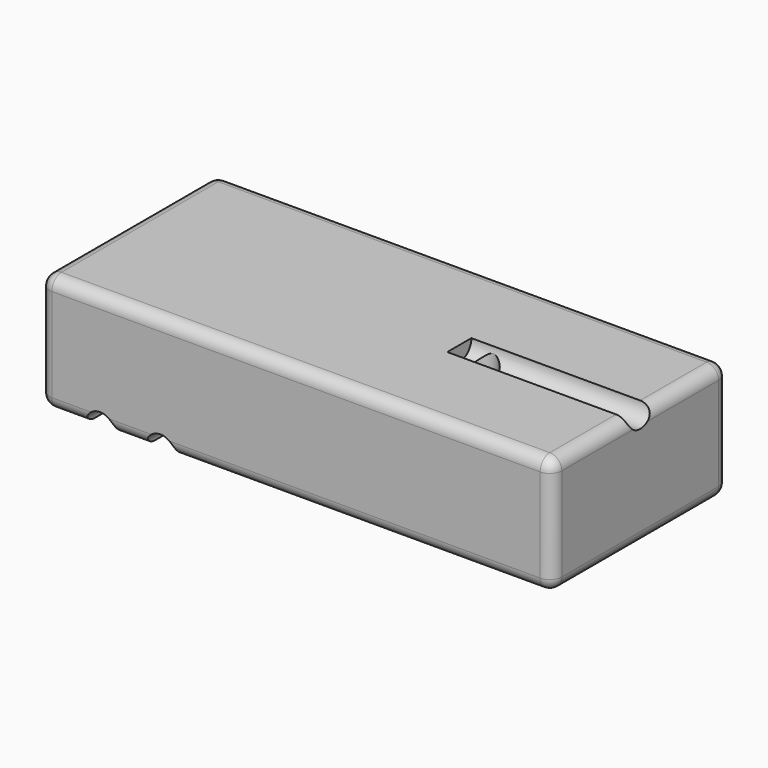
from build123d import *

# Parameters (mm, degrees)
F0_W         = 215.9
F0_H         = 92.71
F1_DEPTH     = 49.53
F3_DEPTH     = 76.2
F5_DEPTH     = 92.71
F6_R         = 5.08
F7_R         = 6.35
F8_DEPTH     = 92.7110001
F9_T1_DEPTH  = 26.67
F9_S5_W      = 5.08
F9_S5_H      = 5.08
F9_T6_DEPTH  = 5.08
F9_S11_W     = 5.08
F9_S11_H     = 5.08
F9_T12_DEPTH = 5.08
F10_R        = 5.588
F11_DEPTH    = 49.5310001


# Not quite as in the source:
# - a fillet or chamfer that OpenCascade refuses, or shapes differently, is made with other operations: its cross-section is extruded or revolved along the edge and cut away or added


with BuildPart() as f1:
    # F0 (on Top) → F1 (new body)
    with BuildSketch(Plane.XY):
        with Locations((107.95, 46.355)):
            Rectangle(F0_W, F0_H)
    extrude(amount=F1_DEPTH)

    # F2 (on face) → F3 (cut)
    with BuildSketch(Plane.YZ.offset(215.9)):
        with BuildLine():
            Line((52.705, 49.53), (40.005, 49.53))
            ThreePointArc((40.005, 49.53), (46.355, 43.18), (52.705, 49.53))
        make_face()
    extrude(amount=-F3_DEPTH, mode=Mode.SUBTRACT)

    # F4 (on face) → F5 (cut, through all)
    with BuildSketch(Plane.XZ):
        with BuildLine():
            Line((19.05, 0), (31.75, 0))
            ThreePointArc((31.75, 0), (25.4, 6.35), (19.05, 0))
        make_face()
    extrude(amount=-F5_DEPTH, mode=Mode.SUBTRACT)

    # F6
    f6_edges = [f1.edges().sort_by_distance(p)[0] for p in [
        (107.95, 0, 49.53),
        (215.9, 20.0025, 49.53),
        (107.95, 92.71, 49.53),
        (215.9, 72.7075, 49.53),
        (0, 92.71, 24.765),
        (0, 46.355, 49.53),
        (0, 0, 24.765),
        (0, 46.355, 0),
        (123.825, 0, 0),
        (123.825, 92.71, 0),
        (215.9, 46.355, 0),
        (215.9, 92.71, 24.765),
        (215.9, 0, 24.765),
    ]]
    fillet(f6_edges, radius=F6_R)

    # F7 (on Front) → F8 (cut, through all)
    with BuildSketch(Plane.XZ):
        with Locations((50.8, 0)):
            Circle(F7_R)
    extrude(amount=-F8_DEPTH, mode=Mode.SUBTRACT)

    # F9: fillet of radius 5.08 on 2 edges, made by hand

    # F9_s2 → F9_t1 (cut)
    with BuildSketch(Plane.YZ.offset(5.08)):
        with BuildLine():
            ThreePointArc((5.08, 0), (1.4878975516, 1.4878975516), (0, 5.08))
            Line((0, 5.08), (0, 0))
            Line((0, 0), (5.08, 0))
        make_face()
        with BuildLine():
            ThreePointArc((92.71, 5.08), (91.2221024484, 1.4878975516), (87.63, 0))
            Line((87.63, 0), (92.71, 0))
            Line((92.71, 0), (92.71, 5.08))
        make_face()
    extrude(amount=F9_T1_DEPTH, mode=Mode.SUBTRACT)


with BuildPart() as f9_tool4:
    # F9_s5 → F9_t6 (new body)
    with BuildSketch(Plane.XZ.offset(-87.63)):
        with Locations((2.54, 2.54)):
            Rectangle(F9_S5_W, F9_S5_H)
    extrude(amount=-F9_T6_DEPTH)

    # F9_s7 → F9_t8 (revolve, cut)
    with BuildSketch(Plane(origin=(5.08, 87.63, 5.08), x_dir=(0.7071067812, 0, 0.7071067812), z_dir=(-0.7071067812, 0, 0.7071067812))):
        with BuildLine():
            ThreePointArc((0, -5.08), (5.08, 0), (0, 5.08))
            Line((0, 5.08), (0, -5.08))
        make_face()
    revolve(axis=Axis((5.08, 87.63, 5.08), (0, 1, 0)), mode=Mode.SUBTRACT)


with BuildPart() as f1_1:
    add(f1.part)

    # F9_t3: cut F9_tool4
    add(f9_tool4.part, mode=Mode.SUBTRACT)


with BuildPart() as f9_tool10:
    # F9_s11 → F9_t12 (new body)
    with BuildSketch(Plane.XY.offset(5.08)):
        with Locations((2.54, 2.54)):
            Rectangle(F9_S11_W, F9_S11_H)
    extrude(amount=-F9_T12_DEPTH)

    # F9_s13 → F9_t14 (revolve, cut)
    with BuildSketch(Plane(origin=(5.08, 5.08, 5.08), x_dir=(0.7071067812, 0.7071067812, 0), z_dir=(-0.7071067812, 0.7071067812, 0))):
        with BuildLine():
            ThreePointArc((0, -5.08), (5.08, 0), (0, 5.08))
            Line((0, 5.08), (0, -5.08))
        make_face()
    revolve(axis=Axis((5.08, 5.08, 5.08), (0, 0, -1)), mode=Mode.SUBTRACT)


with BuildPart() as f1_2:
    add(f1_1.part)

    # F9_t9: cut F9_tool10
    add(f9_tool10.part, mode=Mode.SUBTRACT)

    # F10 (on face) → F11 (cut, through all)
    with BuildSketch(Plane.XY.offset(49.53)):
        with Locations((149.3525841786, 46.6338395569)):
            Circle(F10_R)
    extrude(amount=-F11_DEPTH, mode=Mode.SUBTRACT)


solid = f1_2.part
